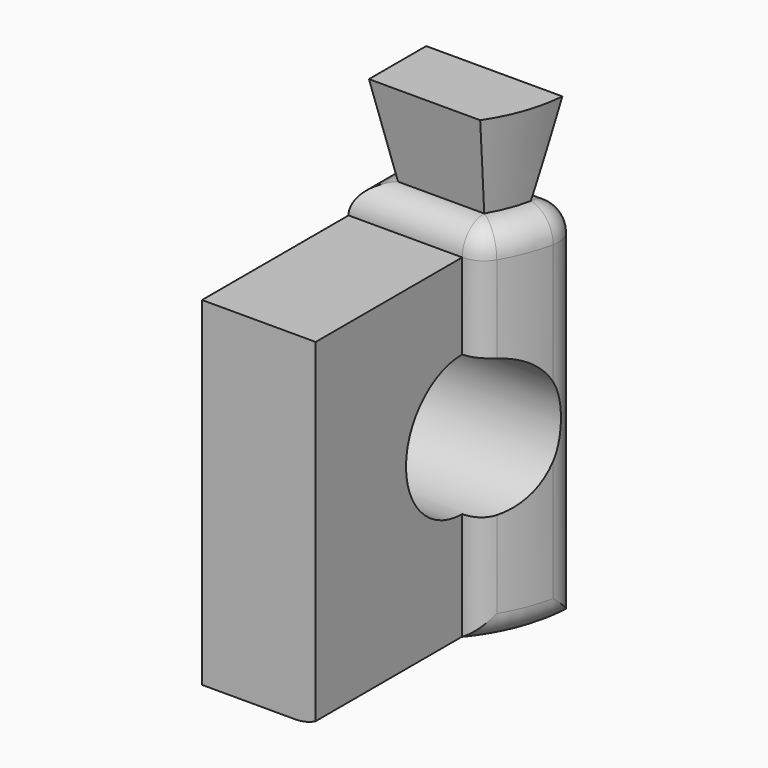
from build123d import *

# Parameters (mm, degrees)
F1_DEPTH               = 50.8
F1_DEPTH_BACK          = 50.8
F2_R                   = 7.62
F3_DEPTH               = 50.8
F4_DEPTH               = 25.4
DRAFT_F4_DRAFTED_ANGLE = -10
F5_R                   = 19.489985333
F6_DEPTH               = 106.68


# Not quite as in the source:
# - an extrude with a draft is written as a straight extrude whose walls are then drafted


with BuildPart() as f1:
    # F0 (on Top) → F1 (new body, two sides)
    with BuildSketch(Plane.XY) as f1_sk:
        with BuildLine():
            ThreePointArc((35.6165115841, -26.1273588985), (41.9787508016, -13.7462453626), (44.1721040979, 0))
            Line((44.1721040979, 0), (0, 0))
            Line((0, 0), (0, -26.1273588985))
            Line((0, -26.1273588985), (35.6165115841, -26.1273588985))
        make_face()
    extrude(amount=F1_DEPTH)
    extrude(f1_sk.sketch, amount=-F1_DEPTH_BACK)

    # F2
    f2_edges = [f1.edges().sort_by_distance(p)[0] for p in [
        (35.616512, -26.127359, 0),
        (41.978751, -13.746245, 50.8),
        (44.172104, 0, 0),
        (41.978751, -13.746245, -50.8),
        (17.808256, -26.127359, 50.8),
        (0, -13.063679, 50.8),
        (22.086052, 0, 50.8),
    ]]
    fillet(f2_edges, radius=F2_R)

    # F3 (add): a face of the model
    f3_faces = [f1.faces().sort_by_distance(p)[0] for p in [
        (15.7476551614, -26.1273588985, -3.7692361525),
    ]]
    extrude(f3_faces, amount=F3_DEPTH)


with BuildPart() as f4_drafted:
    # F4 (new): a face of the model
    f4_faces = [f1.part.faces().sort_by_distance(p)[0] for p in [
        (20.8238277033, -12.9189527173, 50.8),
    ]]
    extrude(f4_faces, amount=F4_DEPTH)

    # draft_F4_drafted
    draft_f4_drafted_walls = [f4_drafted.faces().sort_by_distance(p)[0] for p in [
        (34.072367791, -13.2336717164, 67.7333333333),
        (19.5701870276, -18.5073588985, 67.7333333333),
        (21.6845063847, -7.62, 67.7333333333),
        (7.62, -13.0636794493, 67.7333333333),
    ]]
    draft(draft_f4_drafted_walls, neutral_plane=Plane(origin=(20.8238277033, -12.9189527173, 50.8), x_dir=(1, 0, 0), z_dir=(0, 0, 1)), angle=DRAFT_F4_DRAFTED_ANGLE)


with BuildPart() as f1_1:
    add(f1.part)

    # join_F4_drafted: union F4_drafted
    add(f4_drafted.part)

    # F5 (on face) → F6 (cut)
    with BuildSketch(Plane(origin=(0, 0, 0), x_dir=(0, -1, 0), z_dir=(-1, 0, 0))):
        with Locations((26.1273588985, 0)):
            Circle(F5_R)
    extrude(amount=-F6_DEPTH, mode=Mode.SUBTRACT)


solid = f1_1.part
